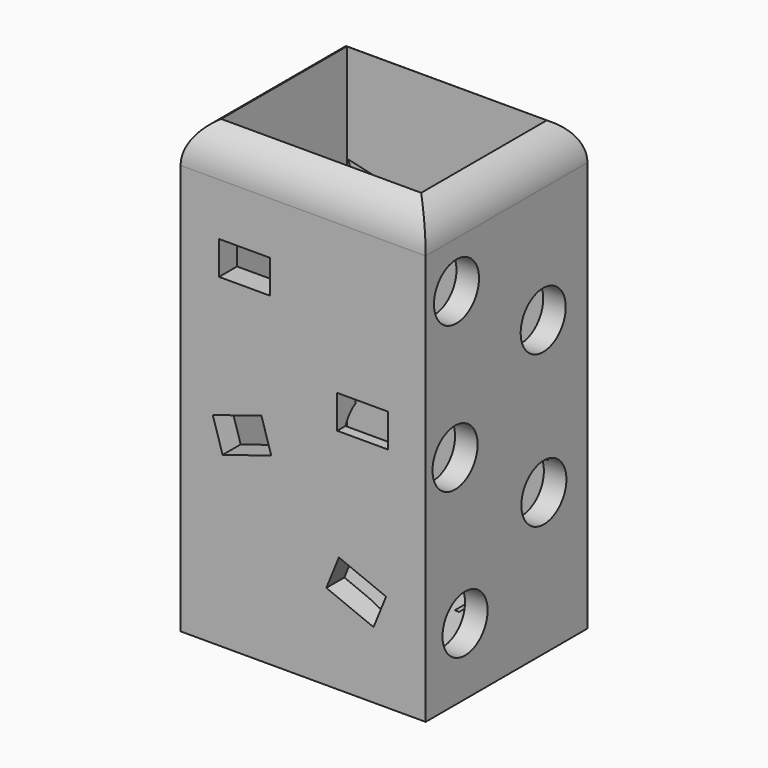
from build123d import *

# Parameters (mm, degrees)
F0_W        = 27.615731582
F0_H        = 22.7759163827
F1_DEPTH    = 51.308
F2_T        = -2.54
F3_T1_DEPTH = 53.015731582
F3_T3_DEPTH = 48.1759163827
F4_W        = 5.7445205748
F4_H        = 3.7603080273
F5_DEPTH    = 4.826
F7_D        = 6.35
F7_DEPTH    = 12.7
F7_TIP      = 1.9077324654
F9_DEPTH    = 8.382


# Not quite as in the source:
# - a fillet or chamfer that OpenCascade refuses, or shapes differently, is made with other operations: its cross-section is extruded or revolved along the edge and cut away or added


with BuildPart() as f1:
    # F0 (on Top) → F1 (new body)
    with BuildSketch(Plane.XY):
        with Locations((-13.807865791, 11.3879581913)):
            Rectangle(F0_W, F0_H)
    extrude(amount=F1_DEPTH)

    # F2
    f2_openings = [f1.faces().sort_by_distance(p)[0] for p in [
        (-13.807866, 11.387958, 51.308),
    ]]
    offset(amount=F2_T, openings=f2_openings)

    # F3: fillet of radius 5.08 on 4 edges, made by hand

    # F3_s2 → F3_t1 (cut)
    with BuildSketch(Plane.YZ.offset(-40.315731582)):
        with BuildLine():
            ThreePointArc((0, 46.228), (1.4878975516, 49.8201024484), (5.08, 51.308))
            Line((5.08, 51.308), (0, 51.308))
            Line((0, 51.308), (0, 46.228))
        make_face()
        with BuildLine():
            ThreePointArc((22.7759163827, 46.228), (21.2880188311, 49.8201024484), (17.6959163827, 51.308))
            Line((17.6959163827, 51.308), (22.7759163827, 51.308))
            Line((22.7759163827, 51.308), (22.7759163827, 46.228))
        make_face()
    extrude(amount=F3_T1_DEPTH, mode=Mode.SUBTRACT)

    # F3_s4 → F3_t3 (cut)
    with BuildSketch(Plane.XZ.offset(-35.4759163827)):
        with BuildLine():
            ThreePointArc((-27.615731582, 46.228), (-26.1278340305, 49.8201024484), (-22.535731582, 51.308))
            Line((-22.535731582, 51.308), (-27.615731582, 51.308))
            Line((-27.615731582, 51.308), (-27.615731582, 46.228))
        make_face()
        with BuildLine():
            ThreePointArc((0, 46.228), (-1.4878975516, 49.8201024484), (-5.08, 51.308))
            Line((-5.08, 51.308), (0, 51.308))
            Line((0, 51.308), (0, 46.228))
        make_face()
    extrude(amount=F3_T3_DEPTH, mode=Mode.SUBTRACT)

    # F4 (on face) → F5 (cut)
    with BuildSketch(Plane.XZ):
        with Locations((-20.4156730324, 38.4546555579)):
            Rectangle(F4_W, F4_H)
        with Locations((-7.0931273513, 27.5189299136)):
            Rectangle(F4_W, F4_H)
        Polygon((-18.5130548821, 24.3505493797), (-23.9980506161, 22.6434060253), (-22.880570963, 19.0529804677), (-17.395575229, 20.7601238221), align=None)
        Polygon((-4.4602522607, 10.9747632246), (-9.781830883, 13.1381673943), (-11.1979744862, 9.6547131094), (-5.8763958639, 7.4913089397), align=None)
    extrude(amount=-F5_DEPTH, mode=Mode.SUBTRACT)

    # F7
    with Locations(Plane.YZ):
        with Locations((4.3385280296, 40.9476608038), (16.5516659617, 33.1388860941), (4.1396417655, 24.540392682), (16.6495069861, 16.0039383918), (5.5445204489, 7.5149172917)):
            Hole(F7_D / 2, depth=F7_DEPTH)
            with Locations((0, 0, -(F7_DEPTH + F7_TIP / 2))):  # 118° drill point
                Cone(0, F7_D / 2, F7_TIP, mode=Mode.SUBTRACT)

    # F8 (on face) → F9 (cut)
    with BuildSketch(Plane(origin=(0, 22.7759163827, 0), x_dir=(-1, 0, 0), z_dir=(0, 1, 0))):
        Polygon((13.0775338039, 35.4098752141), (5.6731416844, 33.7212570012), (11.2572079524, 29.4185951352), align=None)
        Polygon((23.5141057819, 23.2905662243), (15.9249656523, 23.5758839796), (20.2051486408, 17.9745690622), align=None)
        Polygon((7.2458156385, 22.6723130022), (1.6777330699, 17.5077306728), (8.6650072474, 16.573549327), align=None)
        Polygon((23.0783666484, 9.331129957), (15.6739745289, 7.6425117441), (21.258040797, 3.3398498781), align=None)
        Polygon((11.5244448229, 7.3593156172), (3.9536968494, 7.9595066297), (7.997608447, 2.1852989602), align=None)
        Polygon((24.8908895689, 39.4682685534), (17.4864974494, 37.7796503405), (23.0705637174, 33.4769884745), align=None)
        Polygon((10.2386324033, 41.4962964688), (2.6494922737, 41.7816142241), (6.9296752622, 36.1802993067), align=None)
    extrude(amount=-F9_DEPTH, mode=Mode.SUBTRACT)


solid = f1.part
